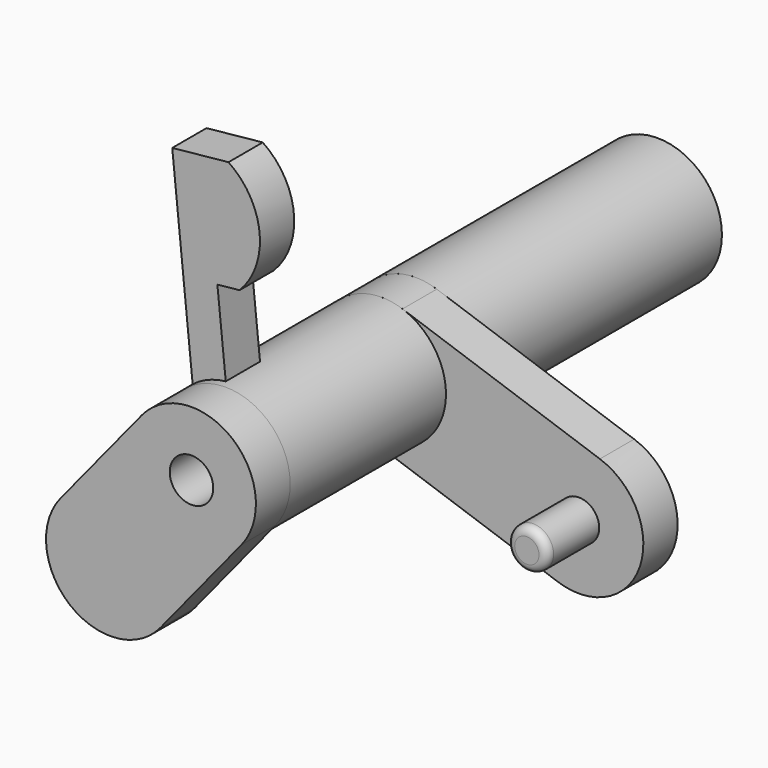
from build123d import *

# Parameters (mm, degrees)
F1_R      = 4.7751995167
F1_R_2    = 1.6129
F2_DEPTH  = 40
F3_R      = 1.6129
F4_DEPTH  = 3.175
F7_DEPTH  = 3.175
F9_R      = 1.6
F9_R_2    = 1.6129
F10_DEPTH = 3.175
F11_R     = 1.5
F12_DEPTH = 8
F13_R     = 0.6
F14_R     = 2.5
F15_DEPTH = 1


# Not quite as in the source:
# - ends of sketch curves that miss each other by under 0.0002 mm in the source are joined


with BuildPart() as f2:
    # F1 (on Front) → F2 (new body)
    with BuildSketch(Plane.XZ):
        with Locations((14.261534, 16.619986)):
            Circle(F1_R)
        with Locations((14.261534, 16.619986)):
            Circle(F1_R_2, mode=Mode.SUBTRACT)
    extrude(amount=-F2_DEPTH)

    # F3 (on Front) → F4 (join)
    with BuildSketch(Plane.XZ):
        with BuildLine():
            Line((10.561823, 19.639037), (4.5555850243, 12.2786630558))
            ThreePointArc((4.5555850243, 12.2786630558), (5.2362451416, 5.5599009071), (11.9550072581, 6.2405613423))
            Line((11.9550072581, 6.2405613423), (17.961245362, 13.600935235))
            ThreePointArc((17.961245362, 13.600935235), (17.2805848408, 20.3196971299), (10.561823, 19.639037))
        make_face()
        with Locations((14.261534, 16.619986)):
            Circle(F3_R, mode=Mode.SUBTRACT)
    extrude(amount=F4_DEPTH)

    # F6 (on offset) → F7 (join)
    with BuildSketch(Plane.XZ.offset(-0.6)):
        with BuildLine():
            Line((9.814391, 35.316965), (11.326905, 20.387013))
            Line((11.326905, 20.387013), (11.451352867, 19.1166915887))
            Line((11.451352867, 19.1166915887), (14.0085988155, 19.1166915887))
            Line((14.0085988155, 19.1166915887), (13.780234, 21.370869))
            Line((13.780234, 21.370869), (13.160689, 27.486366))
            Line((13.160689, 27.486366), (14.803282, 27.652773))
            ThreePointArc((14.803282, 27.652773), (16.2889640924, 31.88808557), (13.984048038, 35.7393820564))
            Line((13.984048038, 35.7393820564), (9.814391, 35.316965))
        make_face()
    extrude(amount=-F7_DEPTH)

    # F9 (on offset) → F10 (join)
    with BuildSketch(Plane.XZ.offset(-17.61)):
        with BuildLine():
            Line((30.4435677445, 16.104987706), (15.814373, 21.135651))
            ThreePointArc((15.814373, 21.135651), (9.7458691018, 18.1728252961), (12.7086947761, 12.104321077))
            Line((12.7086947761, 12.104321077), (27.3378893132, 7.0736583776))
            ThreePointArc((27.3378893132, 7.0736583776), (33.4063931209, 10.036483851), (30.4435677445, 16.104987706))
        make_face()
        with Locations((28.8907284567, 11.5893230666)):
            Circle(F9_R, mode=Mode.SUBTRACT)
        with Locations((14.261534, 16.619986)):
            Circle(F9_R_2, mode=Mode.SUBTRACT)
    extrude(amount=F10_DEPTH)


with BuildPart() as f12:
    # F11 (on face) → F12 (new body)
    with BuildSketch(Plane(origin=(0, 17.61, 0), x_dir=(-1, 0, 0), z_dir=(0, 1, 0))):
        with Locations((-28.8907284567, 11.5893230666)):
            Circle(F11_R)
    extrude(amount=-F12_DEPTH)

    # F13
    f13_edges = [f12.edges().sort_by_distance(p)[0] for p in [
        (30.390728, 9.61, 11.589323),
    ]]
    fillet(f13_edges, radius=F13_R)

    # F14 (on face) → F15 (join)
    with BuildSketch(Plane(origin=(0, 17.61, 0), x_dir=(-1, 0, 0), z_dir=(0, 1, 0))):
        with Locations((-28.8907284567, 11.5893230666)):
            Circle(F14_R)
    extrude(amount=F15_DEPTH)


solid = Compound([f2.part, f12.part])
